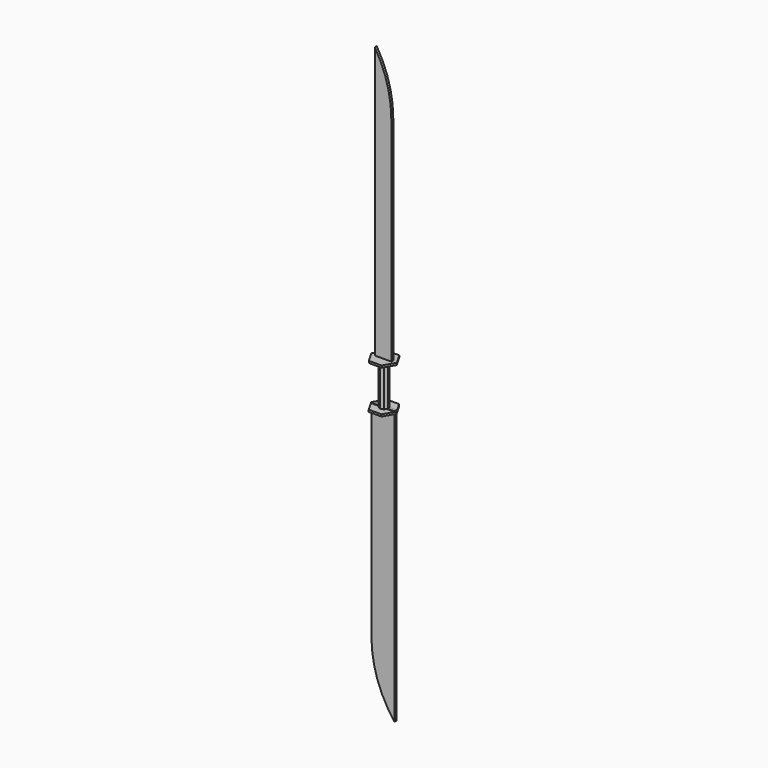
from build123d import *

# Parameters (mm, degrees)
F0_W         = 40.3080582619
F0_H         = 5.9715644456
F1_DEPTH     = 668
F3_DEPTH     = 100
F5_DEPTH     = 5
F6_T1_DEPTH  = 716.1336390313
F9_DEPTH     = 4.9
F10_W        = 56.2156327069
F10_H        = 6.6376542673
F11_DEPTH    = 668
F12_T1_DEPTH = 831.8697028016


# Not quite as in the source:
# - a fillet or chamfer that OpenCascade refuses, or shapes differently, is made with other operations: its cross-section is extruded or revolved along the edge and cut away or added


with BuildPart() as f1:
    # F0 (on Top) → F1 (new body)
    with BuildSketch(Plane.XY):
        Rectangle(F0_W, F0_H)
    extrude(amount=F1_DEPTH)

    # F2 (on Top) → F3 (join)
    with BuildSketch(Plane.XY):
        Polygon((6.5744029718, -8.407556447), (10.5938451005, -1.2962352533), (8.407556447, 6.5744029718), (1.2962352533, 10.5938451005), (-6.5744029718, 8.407556447), (-10.5938451005, 1.2962352533), (-8.407556447, -6.5744029718), (-1.2962352533, -10.5938451005), align=None)
    extrude(amount=-F3_DEPTH)

    # F4 (on Top) → F5 (join)
    with BuildSketch(Plane.XY):
        Polygon((31.1715127681, -0.1368859226), (15.7043030704, 26.9268789703), (-15.4672096977, 27.0637648929), (-31.1715127681, 0.1368859226), (-15.7043030704, -26.9268789703), (15.4672096977, -27.0637648929), align=None)
    extrude(amount=F5_DEPTH)

    # F6: fillet of radius 270.3919189858 on 1 edges, made by hand

    # F6_s2 → F6_t1 (cut)
    with BuildSketch(Plane.XZ.offset(-358.0668195157)):
        with BuildLine():
            ThreePointArc((-20.1540291309, 668), (9.881896476, 599.7882231999), (20.1540291309, 525.9675850829))
            Line((20.1540291309, 525.9675850829), (20.1540291309, 668))
            Line((20.1540291309, 668), (-20.1540291309, 668))
        make_face()
    extrude(amount=F6_T1_DEPTH, mode=Mode.SUBTRACT)

    # F8 (on face) → F9 (join)
    with BuildSketch(Plane(origin=(0, 0, -100), x_dir=(1, 0, 0), z_dir=(0, 0, -1))):
        Polygon((30.9805478901, -0.0372380018), (15.5133381924, 27.0265268911), (-15.6581745757, 27.1634128136), (-31.3624776462, 0.2365338433), (-15.8952679485, -26.8272310495), (15.2762448196, -26.9641169721), align=None)
    extrude(amount=F9_DEPTH)

    # F10 (on offset) → F11 (join)
    with BuildSketch(Plane.XY.offset(-99)):
        Rectangle(F10_W, F10_H)
    extrude(amount=-F11_DEPTH)

    # F12: fillet of radius 270.392 on 1 edges, made by hand

    # F12_s2 → F12_t1 (cut)
    with BuildSketch(Plane.XZ.offset(-415.9348514008)):
        with BuildLine():
            ThreePointArc((-28.1078163534, -601.9535902931), (-13.6683607529, -689.132307188), (28.1078163534, -767))
            Line((28.1078163534, -767), (-28.1078163534, -767))
            Line((-28.1078163534, -767), (-28.1078163534, -601.9535902931))
        make_face()
    extrude(amount=F12_T1_DEPTH, mode=Mode.SUBTRACT)


solid = f1.part
